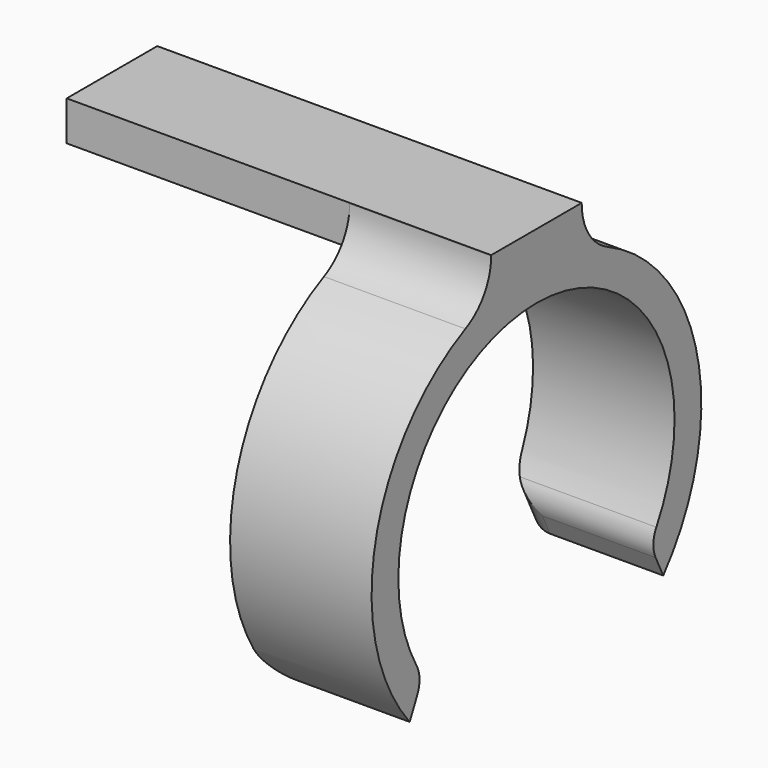
from build123d import *

# Parameters (mm, degrees)
F1_DEPTH = 25
F2_W     = 75
F2_H     = 15
F2_W_2   = 25
F3_DEPTH = 7
F4_R     = 5
F6_W     = 50
F6_H     = 20
F6_W_2   = 25
F7_DEPTH = 7
F8_R     = 10


with BuildPart() as f1:
    # F0 (on Right) → F1 (new body)
    with BuildSketch(Plane.YZ):
        with BuildLine():
            ThreePointArc((-25.1164593902, -17.3035680626), (0, 30.5), (25.1164593902, -17.3035680626))
            Line((25.1164593902, -17.3035680626), (28.0068792885, -23.275158049))
            ThreePointArc((28.0068792885, -23.275158049), (34.7936009681, 10.7481906084), (10, 35.015971637))
            Line((10, 35.015971637), (-10, 35.015971637))
            ThreePointArc((-10, 35.015971637), (-34.7936009681, 10.7481906084), (-28.0068792885, -23.275158049))
            Line((-28.0068792885, -23.275158049), (-25.1164593902, -17.3035680626))
        make_face()
    extrude(amount=F1_DEPTH)

    # F4
    f4_edges = [f1.edges().sort_by_distance(p)[0] for p in [
        (0, -26.561669, -20.289363),
        (12.5, 25.116459, -17.303568),
        (12.5, -25.116459, -17.303568),
        (0, 26.561669, -20.289363),
    ]]
    fillet(f4_edges, radius=F4_R)

    # F6 (on face) → F7 (join)
    with BuildSketch(Plane.XY.offset(35.015971637)):
        with Locations((-25, 0)):
            Rectangle(F6_W, F6_H)
        with Locations((12.5, 0)):
            Rectangle(F6_W_2, F6_H)
    extrude(amount=F7_DEPTH)

    # F8
    f8_edges = [f1.edges().sort_by_distance(p)[0] for p in [
        (12.5, -10, 35.015972),
        (12.5, 10, 35.015972),
    ]]
    fillet(f8_edges, radius=F8_R)


with BuildPart() as f3:
    # F2 (on face) → F3 (new body)
    with BuildSketch(Plane.XY.offset(35.015971637)):
        with Locations((-37.5, 0)):
            Rectangle(F2_W, F2_H)
        with Locations((12.5, 0)):
            Rectangle(F2_W_2, F2_H)
    extrude(amount=F3_DEPTH)


solid = f1.part
